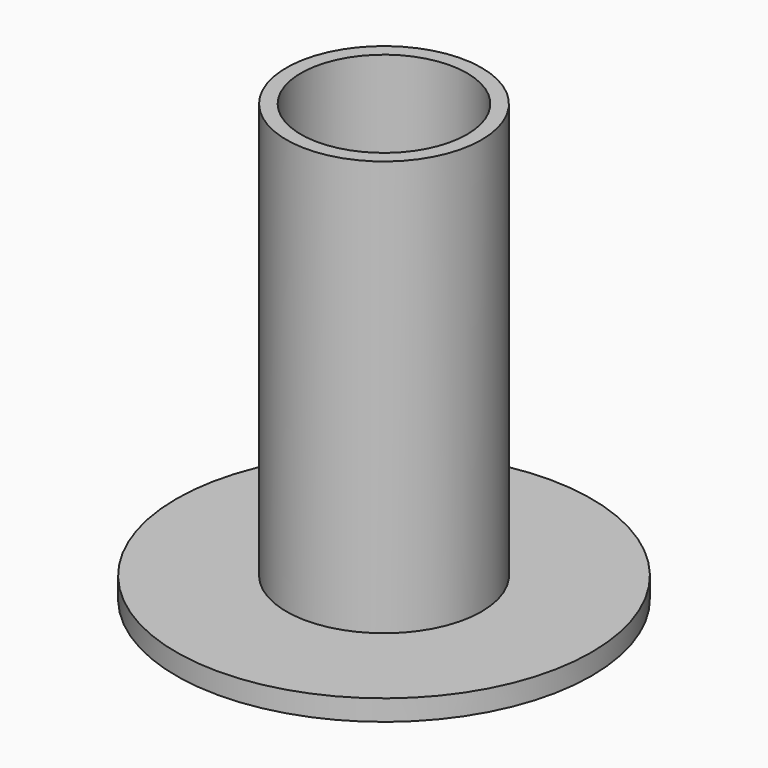
from build123d import *

# Parameters (mm, degrees)
F0_W = 0.7
F0_H = 20


# Not quite as in the source:
# - a feature of the source that left no trace in its solid (it failed there, or was rolled back) is left out


with BuildPart() as f1:
    # F0 (on Front) → F1 (revolve)
    with BuildSketch(Plane.XZ):
        with Locations((4.35, 10)):
            Rectangle(F0_W, F0_H)
        Polygon((4.7, 0), (4, 0), (4, -1), (10, -1), (10, 0), align=None)
    revolve(axis=Axis((0, 0, 8.0465665087), (0, 0, 1)))


solid = f1.part
